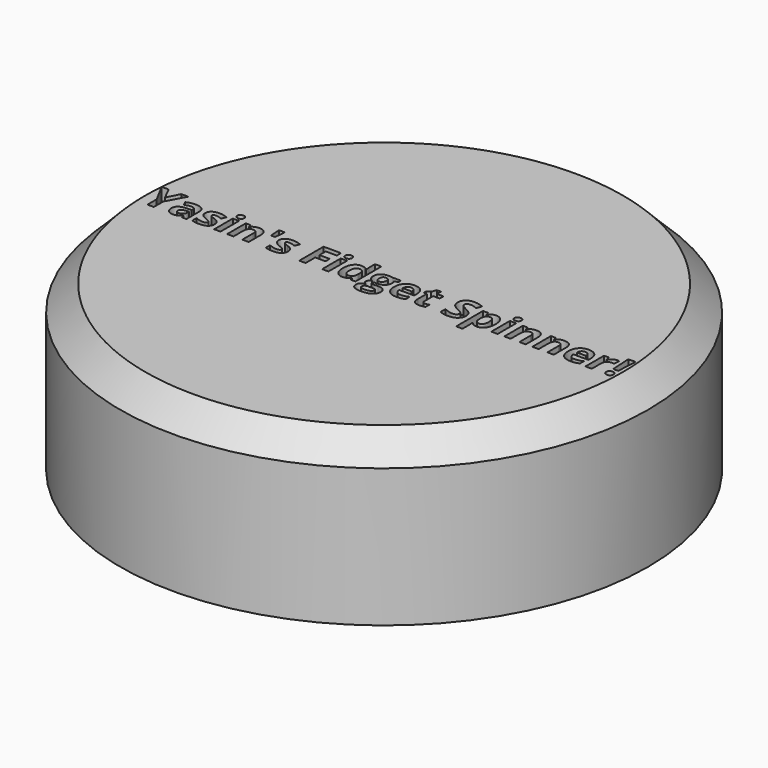
from build123d import *

# Parameters (mm, degrees)
F0_R          = 10.5
F1_DEPTH      = 4
F2_R          = 10
F3_DEPTH      = 2
F4_R          = 4
F4_R_2        = 2.5
F5_DEPTH      = 3
F6_DEPTH      = 5
F8_DEPTH      = 2.5
F7_R          = 1.75
F9_DEPTH      = 7.5
F10_SIZE      = 1
F11_TEXT_SIZE = 1.6944820871
F12_DEPTH     = 0.5


# Not quite as in the source:
# - Text() gives the source's letters only with a copy of the font that has no kerning and outlines rounded to 1/6400 em; it was checked with that copy


with BuildPart() as f1:
    # F0 (on Top) → F1 (new body)
    with BuildSketch(Plane.XY):
        Circle(F0_R)
    extrude(amount=F1_DEPTH)

    # F2 (on face) → F3 (cut)
    with BuildSketch(Plane(origin=(0, 0, 0), x_dir=(1, 0, 0), z_dir=(0, 0, -1))):
        Circle(F2_R)
    extrude(amount=-F3_DEPTH, mode=Mode.SUBTRACT)

    # F4 (on face) → F5 (join)
    with BuildSketch(Plane(origin=(0, 0, 2), x_dir=(1, 0, 0), z_dir=(0, 0, -1))):
        Circle(F4_R)
        Circle(F4_R_2, mode=Mode.SUBTRACT)
    extrude(amount=F5_DEPTH)

    # F6 (add): a face of the model
    f6_faces = [f1.faces().sort_by_distance(p)[0] for p in [
        (0, 0, 2),
    ]]
    extrude(f6_faces, amount=F6_DEPTH)

    # F8 (add): a face of the model
    f8_faces = [f1.faces().sort_by_distance(p)[0] for p in [
        (0, 0, 4),
    ]]
    extrude(f8_faces, amount=F8_DEPTH)

    # F7 (on face) → F9 (cut)
    with BuildSketch(Plane(origin=(0, 0, -3), x_dir=(1, 0, 0), z_dir=(0, 0, -1))):
        Circle(F7_R)
    extrude(amount=-F9_DEPTH, mode=Mode.SUBTRACT)

    # F10
    f10_edges = [f1.edges().sort_by_distance(p)[0] for p in [
        (-10.5, 0, 6.5),
    ]]
    chamfer(f10_edges, length=F10_SIZE)

    # F11 (on face) → F12 (cut)
    with BuildSketch(Plane.XY.offset(6.5)):
        with Locations((-9.4675160297, -0.4350811004)):
            Text("Yasin's Fidget Spinner!", F11_TEXT_SIZE, font='Open Sans', font_style=FontStyle.BOLD, text_align=(TextAlign.LEFT, TextAlign.BOTTOM))
    extrude(amount=-F12_DEPTH, mode=Mode.SUBTRACT)


solid = f1.part
